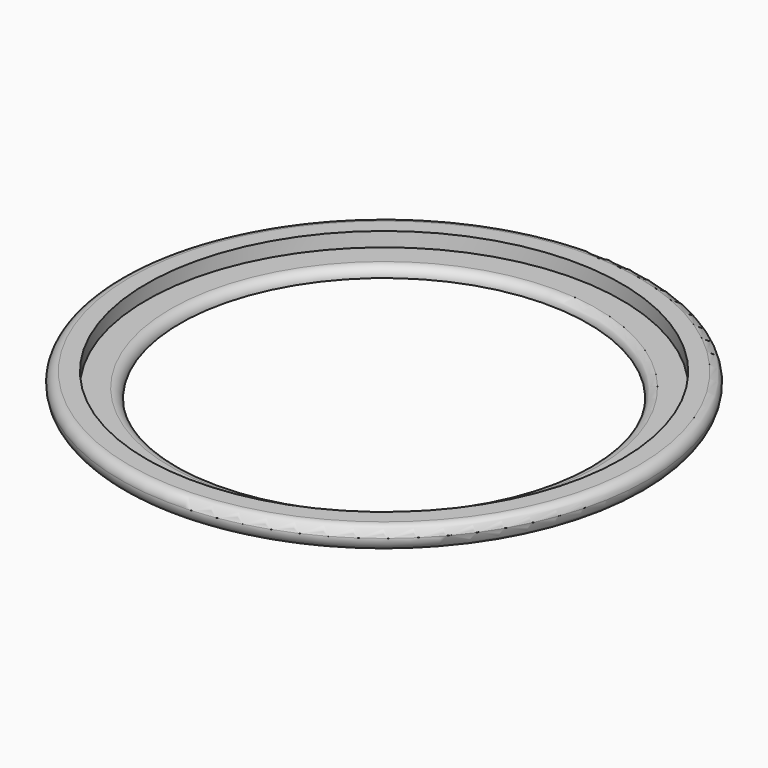
from build123d import *

# Parameters (mm, degrees)
F0_R     = 55
F1_DEPTH = 5
F2_R     = 3
F3_R     = 1.99999
F4_R     = 49.5
F5_DEPTH = 5
F6_R     = 49.5
F6_R_2   = 42.5
F7_DEPTH = 2
F8_R     = 1.99999


# Not quite as in the source:
# - a fillet or chamfer is up to 0.001 mm smaller than in the source, because OpenCascade refuses the exact size


with BuildPart() as f1:
    # F0 (on Top) → F1 (new body)
    with BuildSketch(Plane.XY):
        Circle(F0_R)
    extrude(amount=-F1_DEPTH)

    # F2
    f2_edges = [f1.edges().sort_by_distance(p)[0] for p in [
        (-55, 0, -5),
    ]]
    fillet(f2_edges, radius=F2_R)

    # F3 (radius 2 in the source; OpenCascade refuses exactly that, so slightly less here)
    f3_edges = [f1.edges().sort_by_distance(p)[0] for p in [
        (-55, 0, 0),
    ]]
    fillet(f3_edges, radius=F3_R)

    # F4 (on Top) → F5 (cut)
    with BuildSketch(Plane.XY):
        Circle(F4_R)
    extrude(amount=-F5_DEPTH, mode=Mode.SUBTRACT)

    # F6 (on face) → F7 (join)
    with BuildSketch(Plane(origin=(0, 0, -5), x_dir=(1, 0, 0), z_dir=(0, 0, -1))):
        Circle(F6_R)
        Circle(F6_R_2, mode=Mode.SUBTRACT)
    extrude(amount=-F7_DEPTH)

    # F8 (radius 2 in the source; OpenCascade refuses exactly that, so slightly less here)
    f8_edges = [f1.edges().sort_by_distance(p)[0] for p in [
        (-42.5, 0, -3),
    ]]
    fillet(f8_edges, radius=F8_R)


solid = f1.part
